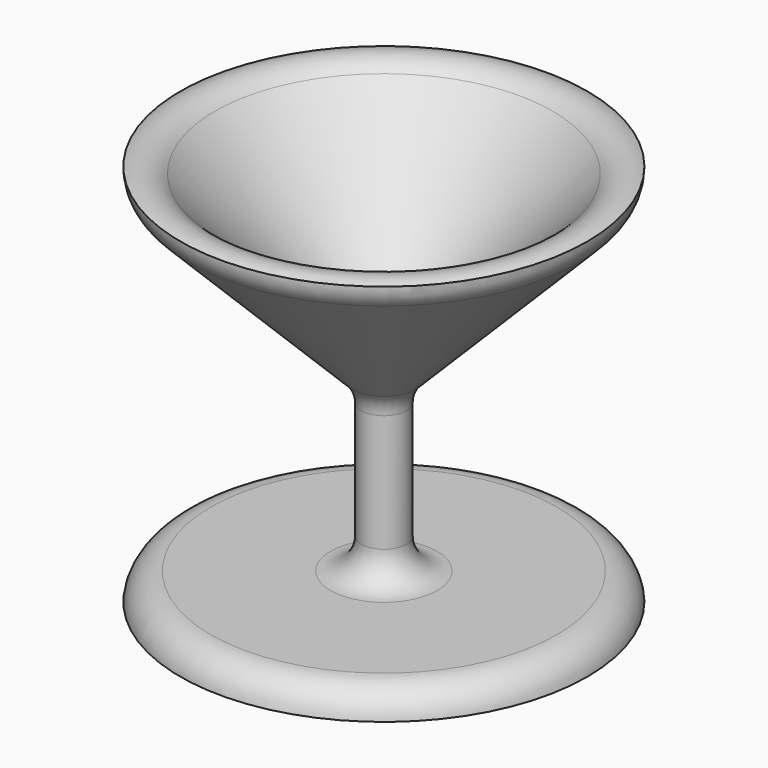
from build123d import *


# Not quite as in the source:
# - a fillet or chamfer that OpenCascade refuses, or shapes differently, is made with other operations: its cross-section is extruded or revolved along the edge and cut away or added


with BuildPart() as f1:
    # F0 (on Front) → F1 (revolve)
    with BuildSketch(Plane.XZ):
        Polygon((0, 20.1451450631), (0, 16.144845517), (2.2029185202, 18.3677908103), (19.8830971494, 36.208700271), (19.8830971494, 40.2089998171), align=None)
        Polygon((0, 2.6437440974), (0, 0), (19.8830971494, 0), (19.8830971494, 2.6437440974), (2.2029185202, 2.6437440974), align=None)
        Polygon((0, 16.144845517), (0, 2.6437440974), (2.2029185202, 2.6437440974), (2.2029185202, 18.3677908103), align=None)
    revolve(axis=Axis((0, 0, 11.3944445803), (0, 0, 1)))

    # F2: fillet of radius 3 on 3 edges, made by hand

    # F2_s1 → F2_t2 (revolve, cut)
    with BuildSketch(Plane.XZ):
        with BuildLine():
            ThreePointArc((19.8830971494, 37.4433964965), (19.6573260634, 36.3016198402), (19.0139945276, 35.331696621))
            Line((19.0139945276, 35.331696621), (19.0566124751, 35.2894626235))
            Line((19.0566124751, 35.2894626235), (19.9430971494, 36.1840063464))
            Line((19.9430971494, 36.1840063464), (19.9430971494, 37.4433964965))
            Line((19.9430971494, 37.4433964965), (19.8830971494, 37.4433964965))
        make_face()
    revolve(axis=Axis((0, 0, 36.208700271), (0, 0, 1)), mode=Mode.SUBTRACT)

    # F2_s3 → F2_t4 (revolve, cut)
    with BuildSketch(Plane.XZ):
        with BuildLine():
            ThreePointArc((19.8830971494, 0), (18.8957107839, 1.8874873657), (16.9043252998, 2.6437440974))
            Line((16.9043252998, 2.6437440974), (16.9043252998, 2.7037440974))
            Line((16.9043252998, 2.7037440974), (19.8830971494, 2.7037440974))
            Line((19.8830971494, 2.7037440974), (19.9430971494, 2.6437440974))
            ThreePointArc((19.9430971494, 2.6437440974), (19.9430971494, 1.3218720487), (19.9426725864, 0.0071251181))
            Line((19.9426725864, 0.0071251181), (19.8830971494, 0))
        make_face()
    revolve(axis=Axis((0, 0, 2.6437440974), (0, 0, 1)), mode=Mode.SUBTRACT)

    # F2_s5 → F2_t6 (revolve)
    with BuildSketch(Plane.XZ):
        with BuildLine():
            ThreePointArc((3.0720211421, 19.2447944602), (2.4286896062, 18.274871241), (2.2029185202, 17.1330945847))
            Line((2.2029185202, 17.1330945847), (2.1429185202, 17.1330945847))
            Line((2.1429185202, 17.1330945847), (2.1429185202, 18.3924847348))
            Line((2.1429185202, 18.3924847348), (3.0294031945, 19.2870284577))
            Line((3.0294031945, 19.2870284577), (3.0720211421, 19.2447944602))
        make_face()
    revolve(axis=Axis((0, 0, 18.3677908103), (0, 0, 1)))

    # F3: fillet of radius 3 on 2 edges, made by hand

    # F3_s1 → F3_t2 (revolve)
    with BuildSketch(Plane.XZ):
        with BuildLine():
            ThreePointArc((2.2029185202, 5.6437440974), (3.0815981766, 3.5224237539), (5.2029185202, 2.6437440974))
            Line((5.2029185202, 2.6437440974), (2.2029185202, 2.6437440974))
            Line((2.2029185202, 2.6437440974), (2.2029185202, 5.6437440974))
        make_face()
    revolve(axis=Axis((0, 0, 2.6437440974), (0, 0, 1)))

    # F3_s3 → F3_t4 (revolve, cut)
    with BuildSketch(Plane.XZ):
        with BuildLine():
            ThreePointArc((19.8830971494, 37.4433827054), (18.1053935902, 37.6561495071), (16.5230757584, 36.8184324094))
            Line((16.5230757584, 36.8184324094), (19.8830971494, 40.2089998171))
            Line((19.8830971494, 40.2089998171), (19.8830971494, 37.4433827054))
        make_face()
    revolve(axis=Axis((0, 0, 40.2089998171), (0, 0, 1)), mode=Mode.SUBTRACT)


solid = f1.part
